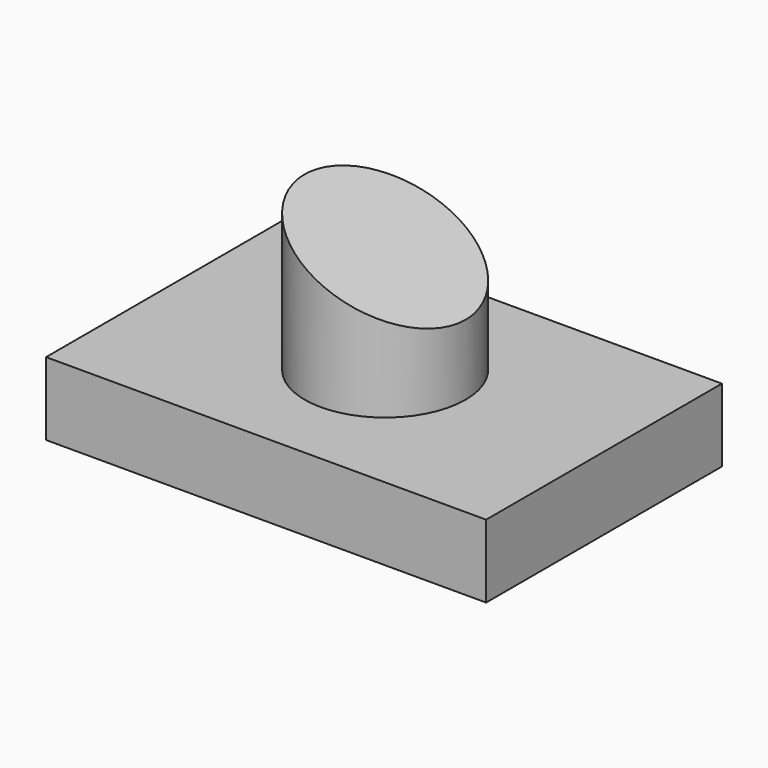
from build123d import *

# Parameters (mm, degrees)
F0_W     = 153.0927270651
F0_H     = 102.5236323476
F1_DEPTH = 25.4
F2_R     = 27.9986216142
F3_DEPTH = 50.8
F5_DEPTH = 121.412


# Not quite as in the source:
# - a feature names something its author has since deleted; it is built from what else it names


with BuildPart() as f1:
    # F0 (on Top) → F1 (new body)
    with BuildSketch(Plane.XY):
        with Locations((-0.1154541969, -0.3463625908)):
            Rectangle(F0_W, F0_H)
    extrude(amount=F1_DEPTH)

    # F2 (on face) → F3 (join)
    with BuildSketch(Plane.XY.offset(25.4)):
        Circle(F2_R)
    extrude(amount=F3_DEPTH)

    # F4 (on face) → F5 (cut)
    with BuildSketch(Plane.XZ.offset(51.6081787646)):
        Polygon((29.090275988, 49.3855252862), (29.2704553796, 77.5817409158), (-30.8739859611, 77.5817409158), align=None)
    extrude(amount=-F5_DEPTH, mode=Mode.SUBTRACT)


solid = f1.part
